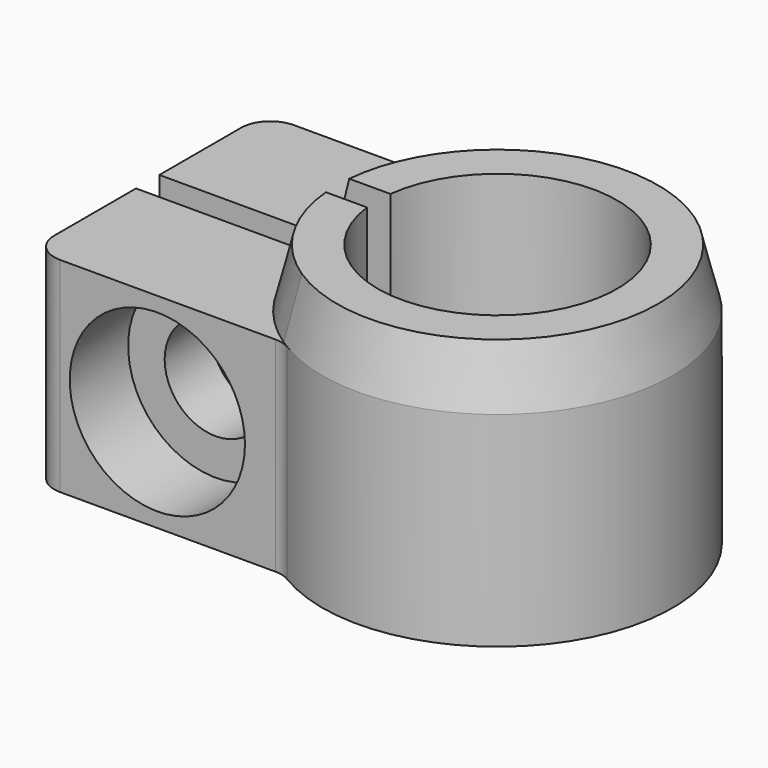
from build123d import *

# Parameters (mm, degrees)
F1_DEPTH       = 9
F2_DEPTH       = 7
F7_D           = 3.5
F7_START       = 4.5
F7_CBORE_D     = 6
F7_CBORE_DEPTH = 2.5
F8_DEPTH       = 6.5
F9_SIZE2       = 1.99999
F9_SIZE        = 0.49999
F10_T1_DEPTH   = 7
F10_T3_DEPTH   = 7


# Not quite as in the source:
# - a fillet or chamfer that OpenCascade refuses, or shapes differently, is made with other operations: its cross-section is extruded or revolved along the edge and cut away or added
# - a fillet or chamfer is up to 0.001 mm smaller than in the source, because OpenCascade refuses the exact size


with BuildPart() as f1:
    # F0 (on Top) → F1 (new body)
    with BuildSketch(Plane.XY):
        with BuildLine():
            ThreePointArc((-4.0693979899, 0.5), (4.1, 0), (-4.0693979899, -0.5))
            Line((-4.0693979899, -0.5), (-5.9791303716, -0.5))
            ThreePointArc((-5.9791303716, -0.5), (-5.1638421749, -3.0552796914), (-3.3166247904, -5))
            ThreePointArc((-3.3166247904, -5), (6, 0), (-3.3166247904, 5))
            ThreePointArc((-3.3166247904, 5), (-5.1638421749, 3.0552796914), (-5.9791303716, 0.5))
            Line((-5.9791303716, 0.5), (-4.0693979899, 0.5))
        make_face()
    extrude(amount=F1_DEPTH)

    # F0 (on Top) → F2 (join)
    with BuildSketch(Plane.XY):
        with BuildLine():
            Line((-11.9791303716, 0.5), (-5.9791303716, 0.5))
            ThreePointArc((-5.9791303716, 0.5), (-5.1638421749, 3.0552796914), (-3.3166247904, 5))
            Line((-3.3166247904, 5), (-11.9791303716, 5))
            Line((-11.9791303716, 5), (-11.9791303716, 0.5))
        make_face()
        with BuildLine():
            ThreePointArc((-3.3166247904, -5), (-5.1638421749, -3.0552796914), (-5.9791303716, -0.5))
            Line((-5.9791303716, -0.5), (-11.9791303716, -0.5))
            Line((-11.9791303716, -0.5), (-11.9791303716, -5))
            Line((-11.9791303716, -5), (-3.3166247904, -5))
        make_face()
    extrude(amount=F2_DEPTH)

    # F7 (through all)
    # its depths count from where the whole tool has entered the part; down to there all is cleared
    with Locations(Plane.XZ.offset(9.5).offset(-F7_START)):
        with Locations((-7.647877581, 3.5)):
            CounterBoreHole(F7_D / 2, F7_CBORE_D / 2, F7_CBORE_DEPTH)

    # F6 (on offset) → F8 (cut)
    with BuildSketch(Plane(origin=(0, 9.5, 0), x_dir=(-1, 0, 0), z_dir=(0, 1, 0))):
        Polygon((6.0024293138, 0.65), (9.2933258481, 0.65), (10.9387741153, 3.5), (9.2933258481, 6.35), (6.0024293138, 6.35), (4.3569810466, 3.5), align=None)
    extrude(amount=-F8_DEPTH, mode=Mode.SUBTRACT)

    # F9 (size 0.5 and 2 in the source; OpenCascade refuses exactly that, so slightly less here)
    f9_edges = [f1.edges().sort_by_distance(p)[0] for p in [
        (5.400488, -2.614332, 9),
    ]]
    f9_side = f1.faces().sort_by_distance((-5.017914, 2.968938, 9))[0]
    chamfer(f9_edges, length=F9_SIZE, length2=F9_SIZE2, reference=f9_side)

    # F10: fillet of radius 1 on 4 edges, made by hand

    # F10_s2 → F10_t1 (join)
    with BuildSketch(Plane.XY):
        with BuildLine():
            ThreePointArc((-3.0904725218, -5.1428571429), (-3.3382900336, -5.0363758883), (-3.6055512755, -5))
            Line((-3.6055512755, -5), (-3.6055512755, -4.98))
            Line((-3.6055512755, -4.98), (-3.3166247904, -4.98))
            Line((-3.3166247904, -4.98), (-3.3055693744, -4.9833333333))
            ThreePointArc((-3.3055693744, -4.9833333333), (-3.1936637184, -5.0557800638), (-3.0801709468, -5.1257142857))
            Line((-3.0801709468, -5.1257142857), (-3.0904725218, -5.1428571429))
        make_face()
        with BuildLine():
            ThreePointArc((-3.0904725218, 5.1428571429), (-3.3382900336, 5.0363758883), (-3.6055512755, 5))
            Line((-3.6055512755, 5), (-3.6055512755, 4.98))
            Line((-3.6055512755, 4.98), (-3.3166247904, 4.98))
            Line((-3.3166247904, 4.98), (-3.3055693744, 4.9833333333))
            ThreePointArc((-3.3055693744, 4.9833333333), (-3.1936637184, 5.0557800638), (-3.0801709468, 5.1257142857))
            Line((-3.0801709468, 5.1257142857), (-3.0904725218, 5.1428571429))
        make_face()
    extrude(amount=F10_T1_DEPTH)

    # F10_s4 → F10_t3 (cut)
    with BuildSketch(Plane.XY):
        with BuildLine():
            ThreePointArc((-10.9791303716, -5), (-11.6862371527, -4.7071067812), (-11.9791303716, -4))
            Line((-11.9791303716, -4), (-11.9991303716, -4))
            Line((-11.9991303716, -4), (-11.9991303716, -5.02))
            Line((-11.9991303716, -5.02), (-10.9791303716, -5.02))
            Line((-10.9791303716, -5.02), (-10.9791303716, -5))
        make_face()
        with BuildLine():
            ThreePointArc((-11.9791303716, 4), (-11.6862371527, 4.7071067812), (-10.9791303716, 5))
            Line((-10.9791303716, 5), (-10.9791303716, 5.02))
            Line((-10.9791303716, 5.02), (-11.9991303716, 5.02))
            Line((-11.9991303716, 5.02), (-11.9991303716, 4))
            Line((-11.9991303716, 4), (-11.9791303716, 4))
        make_face()
    extrude(amount=F10_T3_DEPTH, mode=Mode.SUBTRACT)


solid = f1.part
